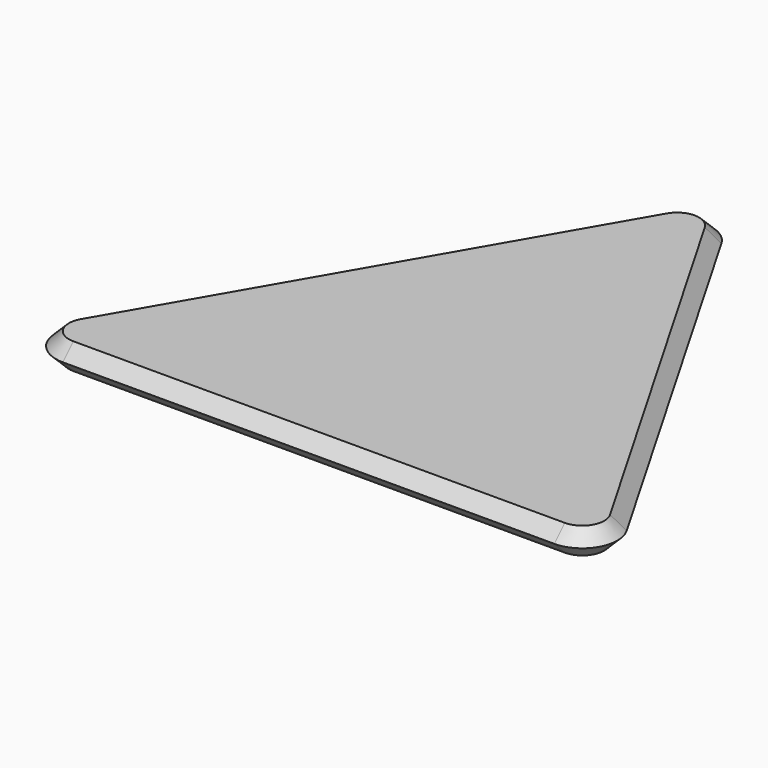
from build123d import *

# Parameters (mm, degrees)
F1_DEPTH = 0.75
F2_SIZE  = 0.74999


# Not quite as in the source:
# - a fillet or chamfer is up to 0.001 mm smaller than in the source, because OpenCascade refuses the exact size


with BuildPart() as f1:
    # F0 (on Top) → F1 (new body, symmetric)
    with BuildSketch(Plane.XY):
        with BuildLine():
            ThreePointArc((1.7320508076, 27.3108891325), (0, 28.3108891325), (-1.7320508076, 27.3108891325))
            Line((-1.7320508076, 27.3108891325), (-15.7679491924, 3))
            ThreePointArc((-15.7679491924, 3), (-15.7679491924, 1), (-14.0358983849, 0))
            Line((-14.0358983849, 0), (14.0358983849, 0))
            ThreePointArc((14.0358983849, 0), (15.7679491924, 1), (15.7679491924, 3))
            Line((15.7679491924, 3), (1.7320508076, 27.3108891325))
        make_face()
    extrude(amount=F1_DEPTH, both=True)

    # F2 (size 0.75 in the source; OpenCascade refuses exactly that, so slightly less here)
    f2_edges = [f1.edges().sort_by_distance(p)[0] for p in [
        (8.75, 15.155445, 0.75),
        (8.75, 15.155445, -0.75),
        (0, 0, 0.75),
        (-8.75, 15.155445, 0.75),
        (0, 0, -0.75),
        (-8.75, 15.155445, -0.75),
    ]]
    chamfer(f2_edges, length=F2_SIZE)


solid = f1.part
